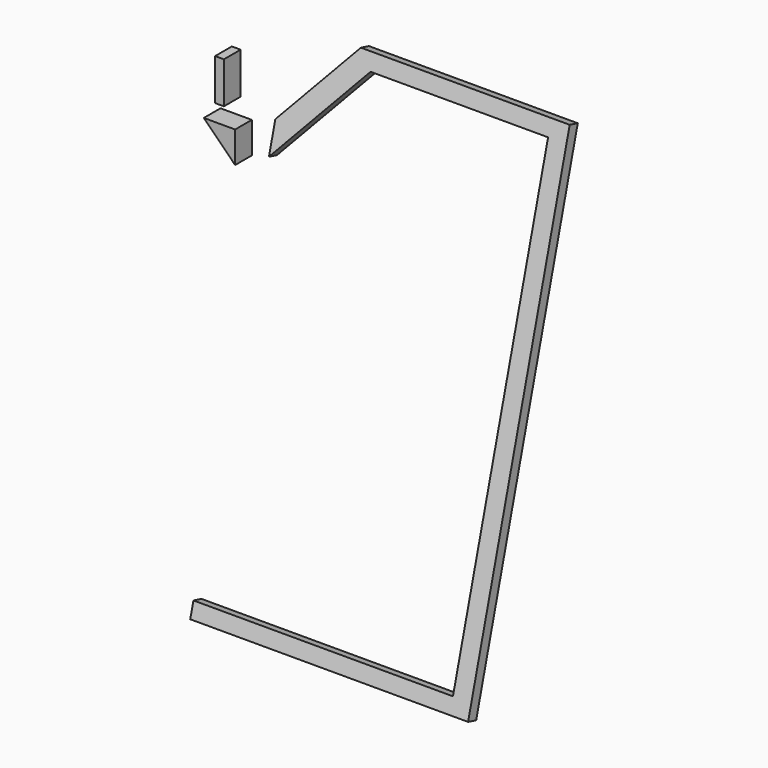
from build123d import *

# Parameters (mm, degrees)
F1_DEPTH     = 1.27
F2_ANGLE     = -15
F3_TEXT_SIZE = 14.1111111111
F4_DEPTH     = 5.08


# Not quite as in the source:
# - Text() gives the source's letters only with a copy of the font that has no kerning and outlines rounded to 1/6400 em; it was checked with that copy


with BuildPart() as f1:
    # F0 (on Front) → F1 (new body, symmetric)
    with BuildSketch(Plane.XZ):
        Polygon((0, 47.2412850702), (0, 39.7365093231), (19.9515821857, 62.779182091), (63.1315821857, 62.779182091), (63.1315821857, -48.980817909), (0, -48.980817909), (0, -52.7444653501), (67.592581673, -52.7444653501), (67.592581673, 66.6355346499), (16.792581673, 66.6355346499), align=None)
    extrude(amount=F1_DEPTH, both=True)


with BuildPart() as f1_1:
    # F2: moved
    add(f1.part.rotate(Axis((33.7962908365, 1.27, -52.7444653501), (1, 0, 0)), F2_ANGLE))


with BuildPart() as f4:
    # F3 (on Front) → F4 (new body)
    with BuildSketch(Plane.XZ):
        Polygon((14.0372590157, 58.9511548834), (6.4172590157, 58.9511548834), (14.0372590157, 51.3311548834), align=None)
        with Locations((7.9026819895, 63.0188968002)):
            Text('I', F3_TEXT_SIZE, font='Open Sans', font_style=FontStyle.BOLD, text_align=(TextAlign.LEFT, TextAlign.BOTTOM))
    extrude(amount=F4_DEPTH)


solid = Compound([f1_1.part, f4.part])
